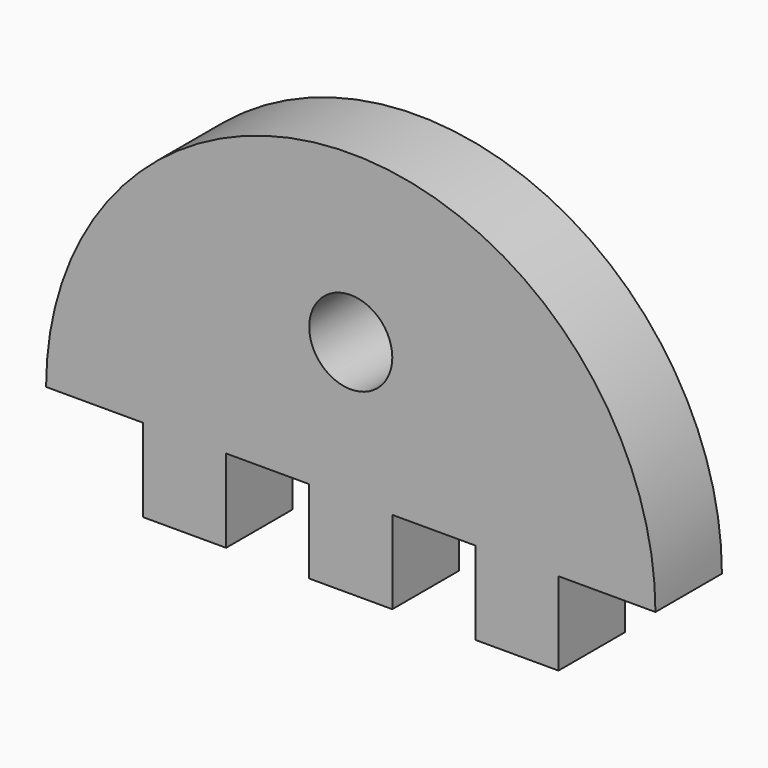
from build123d import *

# Parameters (mm, degrees)
F0_R     = 1.5
F1_DEPTH = 3


# Not quite as in the source:
# - a feature names something its author has since deleted; it is built from what else it names


with BuildPart() as f1:
    # F0 (on Front) → F1 (new body)
    with BuildSketch(Plane.XZ):
        with BuildLine():
            Line((7.5, 0), (11, 0))
            ThreePointArc((11, 0), (0, 11), (-11, 0))
            Line((-11, 0), (-7.5, 0))
            Line((-7.5, 0), (-7.5, -3))
            Line((-7.5, -3), (-4.5, -3))
            Line((-4.5, -3), (-4.5, 0))
            Line((-4.5, 0), (-1.5, 0))
            Line((-1.5, 0), (-1.5, -3))
            Line((-1.5, -3), (1.5, -3))
            Line((1.5, -3), (1.5, 0))
            Line((1.5, 0), (4.5, 0))
            Line((4.5, 0), (4.5, -3))
            Line((4.5, -3), (7.5, -3))
            Line((7.5, -3), (7.5, 0))
        make_face()
        with Locations((0, 5)):
            Circle(F0_R, mode=Mode.SUBTRACT)
    extrude(amount=F1_DEPTH)


solid = f1.part
